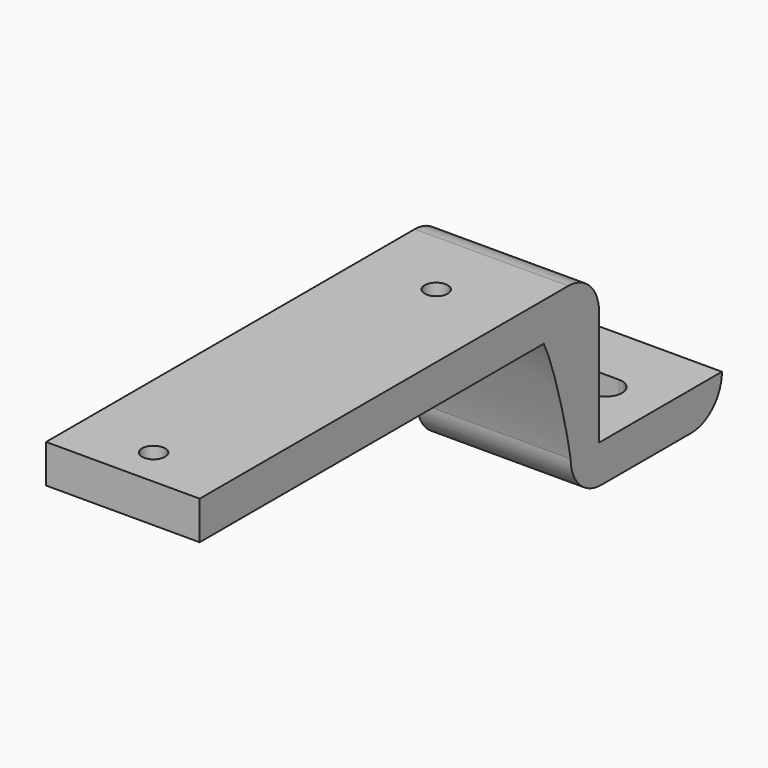
from build123d import *

# Parameters (mm, degrees)
F1_DEPTH = 20
F2_R     = 1.5
F3_DEPTH = 5
F4_W     = 10
F4_H     = 4.2
F5_DEPTH = 5
F6_R     = 2.09999
F7_R     = 4.999


# Not quite as in the source:
# - a fillet or chamfer is up to 0.001 mm smaller than in the source, because OpenCascade refuses the exact size


with BuildPart() as f1:
    # F0 (on Right) → F1 (new body)
    with BuildSketch(Plane.YZ):
        with BuildLine():
            Line((76.2121204979, -15), (56.2121204979, -15))
            Line((56.2121204979, -15), (51.5942049014, -15))
            add(Edge.make_bspline(
                [(51.5942049014, -15), (51.5942049014, -16.6666666667), (51.5942043035, -18.3333333333), (51.5942049014, -20)],
                knots=[0, 0, 0, 0, 5, 5, 5, 5], degree=3))
            Line((51.5942049014, -20), (76.2121204979, -20))
            Line((76.2121204979, -20), (76.2121204979, -15))
        make_face()
        with BuildLine():
            Line((56.2121204979, -15), (56.2121204979, 0))
            Line((56.2121204979, 0), (47.2121204979, 0))
            add(Edge.make_bspline(
                [(47.2121204979, 0), (48.878788136, -3.0912153851), (50.9981620768, -11.3440190259), (51.5942049014, -15)],
                knots=[0, 0, 0, 0, 15.6269851129, 15.6269851129, 15.6269851129, 15.6269851129], degree=3))
            Line((51.5942049014, -15), (56.2121204979, -15))
        make_face()
        Polygon((56.2121204979, 0), (56.2121204979, 5), (-8.7878795021, 5), (-8.7878795021, 0), (47.2121204979, 0), align=None)
    extrude(amount=F1_DEPTH)

    # F2 (on face) → F3 (cut)
    with BuildSketch(Plane(origin=(0, 0, 0), x_dir=(1, 0, 0), z_dir=(0, 0, -1))):
        with Locations((10, -42.2121204979)):
            Circle(F2_R)
        with Locations((10, 3.7878795021)):
            Circle(F2_R)
    extrude(amount=-F3_DEPTH, mode=Mode.SUBTRACT)

    # F4 (on face) → F5 (cut)
    with BuildSketch(Plane.XY.offset(-15)):
        with Locations((10, 66.2121204979)):
            Rectangle(F4_W, F4_H)
    extrude(amount=-F5_DEPTH, mode=Mode.SUBTRACT)

    # F6 (radius 2.1 in the source; OpenCascade refuses exactly that, so slightly less here)
    f6_edges = [f1.edges().sort_by_distance(p)[0] for p in [
        (5, 68.31212, -17.5),
        (15, 68.31212, -17.5),
        (15, 64.11212, -17.5),
        (5, 64.11212, -17.5),
    ]]
    fillet(f6_edges, radius=F6_R)

    # F7 (radius 5 in the source; OpenCascade refuses exactly that, so slightly less here)
    f7_edges = [f1.edges().sort_by_distance(p)[0] for p in [
        (10, 56.21212, 5),
        (10, 76.21212, -20),
        (10, 51.594205, -20),
    ]]
    fillet(f7_edges, radius=F7_R)


solid = f1.part
